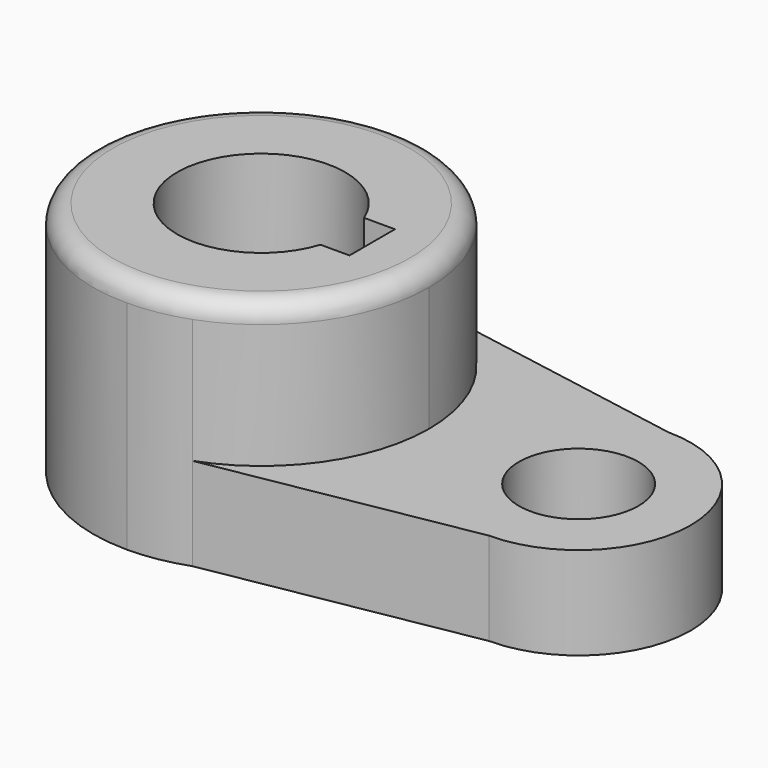
from build123d import *

# Parameters (mm, degrees)
F0_R     = 14.2875
F1_DEPTH = 40.2336
F0_R_2   = 10.16
F2_DEPTH = 15.7734
F4_DEPTH = 40.2336


# Not quite as in the source:
# - a fillet or chamfer that OpenCascade refuses, or shapes differently, is made with other operations: its cross-section is extruded or revolved along the edge and cut away or added


with BuildPart() as f1:
    # F0 (on Top) → F1 (new body)
    with BuildSketch(Plane.XY):
        with BuildLine():
            ThreePointArc((9.780704698, 26.8489932886), (4.9659159165, 28.1401901932), (0, 28.575))
            Line((0, 28.575), (9.780704698, 26.8489932886))
        make_face()
        with BuildLine():
            Line((9.780704698, -26.8489932886), (0, -28.575))
            ThreePointArc((0, -28.575), (4.9659159165, -28.1401901932), (9.780704698, -26.8489932886))
        make_face()
        with BuildLine():
            Line((9.780704698, 26.8489932886), (0, 28.575))
            ThreePointArc((0, 28.575), (-28.575, 0), (0, -28.575))
            Line((0, -28.575), (9.780704698, -26.8489932886))
            ThreePointArc((9.780704698, -26.8489932886), (23.4095521288, -16.3866864902), (28.575, 0))
            ThreePointArc((28.575, 0), (23.4095521288, 16.3866864902), (9.780704698, 26.8489932886))
        make_face()
        Circle(F0_R, mode=Mode.SUBTRACT)
    extrude(amount=F1_DEPTH)

    # F0 (on Top) → F2 (join)
    with BuildSketch(Plane.XY):
        with BuildLine():
            Line((53.975, 19.05), (9.780704698, 26.8489932886))
            ThreePointArc((9.780704698, 26.8489932886), (23.4095521288, 16.3866864902), (28.575, 0))
            ThreePointArc((28.575, 0), (23.4095521288, -16.3866864902), (9.780704698, -26.8489932886))
            Line((9.780704698, -26.8489932886), (53.975, -19.05))
            ThreePointArc((53.975, -19.05), (73.025, 0), (53.975, 19.05))
        make_face()
        with Locations((53.975, 0)):
            Circle(F0_R_2, mode=Mode.SUBTRACT)
    extrude(amount=F2_DEPTH)

    # F3 (on face) → F4 (cut, through all)
    with BuildSketch(Plane.XY.offset(40.2336)):
        with BuildLine():
            Line((18.5357414117, 5.2549776766), (13.2860026294, 5.2549776766))
            ThreePointArc((13.2860026294, 5.2549776766), (14.0348925685, 2.6747797744), (14.2875, 0))
            ThreePointArc((14.2875, 0), (14.1130788652, -2.2256821862), (13.5940741111, -4.3970223234))
            Line((13.5940741111, -4.3970223234), (18.5357414117, -4.3970223234))
            Line((18.5357414117, -4.3970223234), (18.5357414117, 5.2549776766))
        make_face()
    extrude(amount=-F4_DEPTH, mode=Mode.SUBTRACT)

    # F5: fillet of radius 3.302 on 1 edges, made by hand

    # F5_s1 → F5_t2 (revolve, cut)
    with BuildSketch(Plane.YZ):
        with BuildLine():
            ThreePointArc((28.575, 36.9316), (27.6078665915, 39.2664665915), (25.273, 40.2336))
            Line((25.273, 40.2336), (28.575, 40.2336))
            Line((28.575, 40.2336), (28.575, 36.9316))
        make_face()
    revolve(axis=Axis((0, 0, 40.2336), (0, 0, 1)), mode=Mode.SUBTRACT)


solid = f1.part
